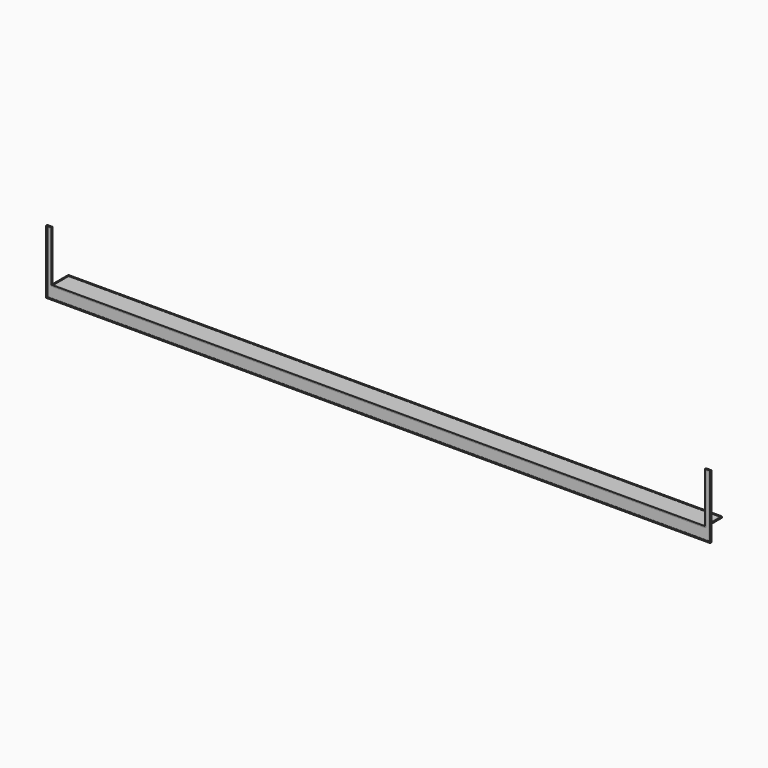
from build123d import *

# Parameters (mm, degrees)
F1_DEPTH     = 3.175
F3_W         = 1562.1
F3_H         = 50.8
F4_DEPTH     = 3.175
F5_T         = 2.54
F5_T3_DEPTH  = 8.255
F5_T5_DEPTH  = 1567.18
F6_T         = 2.54
F6_T3_DEPTH  = 8.255
F6_T5_DEPTH  = 8.255
F6_T7_DEPTH  = 1567.18
F6_T9_DEPTH  = 5.715
F6_T11_DEPTH = 50.165
F6_T13_DEPTH = 5.715
F6_T15_DEPTH = 1562.1


# Not quite as in the source:
# - a shell that OpenCascade refuses in one call is made with other operations: the cavity is built on its own and cut out


with BuildPart() as f1:
    # F0 (on Front) → F1 (new body)
    with BuildSketch(Plane.XZ):
        Polygon((-781.05, 156.1854919385), (-793.75, 156.1854919385), (-793.75, 3.7854919385), (793.75, 3.7854919385), (793.75, 156.1854919385), (781.05, 156.1854919385), (781.05, 35.5354919385), (-781.05, 35.5354919385), align=None)
    extrude(amount=F1_DEPTH)

    # F3 (on face) → F4 (join)
    with BuildSketch(Plane.XY.offset(35.5354919385)):
        with Locations((0, 22.225)):
            Rectangle(F3_W, F3_H)
    extrude(amount=-F4_DEPTH)

    # F5: shell of thickness 2.54, made by hand


with BuildPart() as f5_core1:
    # F5_t2: copy of F1
    add(f1.part)

    # the walls: a layer under each face that stays
    f5_faces = [f5_core1.faces().sort_by_distance(p)[0] for p in [
        (-781.05, -1.5875, 95.8604919385),
        (-787.4, -1.5875, 156.1854919385),
        (-529.1666666667, 0, 29.1854919385),
        (-529.1666666667, -3.175, 29.1854919385),
        (781.05, -1.5875, 95.8604919385),
        (-793.75, -1.5875, 79.9854919385),
        (-781.05, 23.8125, 33.9479919385),
        (0, 23.8125, 32.3604919385),
        (781.05, 23.8125, 33.9479919385),
        (787.4, -1.5875, 156.1854919385),
        (793.75, -1.5875, 79.9854919385),
        (0, -1.5875, 3.7854919385),
        (0, 47.625, 33.9479919385),
    ]]
    thicken(f5_faces, amount=-F5_T, mode=Mode.SUBTRACT)

    # F5_s4 → F5_t3 (cut)
    with BuildSketch(Plane.XY.offset(29.8204919385)):
        Polygon((-781.0754, 0.0254), (-781.05, -2.54), (-778.51, -2.54), (-778.51, 0), align=None)
        Polygon((781.0754, 0.0254), (781.05, -2.54), (778.51, -2.54), (778.51, 0), align=None)
    extrude(amount=F5_T3_DEPTH, mode=Mode.SUBTRACT)

    # F5_s6 → F5_t5 (cut)
    with BuildSketch(Plane.YZ.offset(-783.59)):
        Polygon((0.0254, 32.3350919385), (-2.54, 32.3604919385), (-2.54, 34.9004919385), (0, 34.9004919385), align=None)
    extrude(amount=F5_T5_DEPTH, mode=Mode.SUBTRACT)


with BuildPart() as f1_1:
    add(f1.part)

    # what is left inside the walls is the cavity
    f5_cavity = [f5_core1.part.solids().sort_by_distance(p)[0] for p in [
        (0, 14.605, 34.925892),
    ]]
    add(f5_cavity, mode=Mode.SUBTRACT)

    # F6: shell of thickness 2.54, made by hand


with BuildPart() as f6_core1:
    # F6_t2: copy of F1
    add(f1_1.part)

    # the walls: a layer under each face that stays
    f6_faces = [f6_core1.faces().sort_by_distance(p)[0] for p in [
        (-781.05, -1.5875, 95.8604919385),
        (728.98, -1.4816666667, 35.5354919385),
        (-787.4, -1.5875, 156.1854919385),
        (-529.1666666667, 0, 29.1854919385),
        (781.05, -1.5875, 95.8604919385),
        (781.05, 23.8125, 33.9479919385),
        (0, 47.625, 33.9479919385),
        (-781.05, 23.8125, 33.9479919385),
        (778.51, 22.225, 35.2179919385),
        (0, -0.635, 35.2179919385),
        (-778.51, 22.225, 35.2179919385),
        (0, 45.085, 35.2179919385),
        (-793.75, -1.5875, 79.9854919385),
        (0, 23.8125, 32.3604919385),
        (787.4, -1.5875, 156.1854919385),
        (793.75, -1.5875, 79.9854919385),
        (0, -1.5875, 3.7854919385),
        (0, 22.225, 34.9004919385),
    ]]
    thicken(f6_faces, amount=-F6_T, mode=Mode.SUBTRACT)

    # F6_s4 → F6_t3 (cut)
    with BuildSketch(Plane.XZ.offset(-2.54)):
        Polygon((-781.0246, 35.5608919385), (-783.59, 35.5354919385), (-783.59, 32.9954919385), (-781.05, 32.9954919385), align=None)
        Polygon((781.0246, 35.5608919385), (781.05, 32.9954919385), (783.59, 32.9954919385), (783.59, 35.5354919385), align=None)
    extrude(amount=F6_T3_DEPTH, mode=Mode.SUBTRACT)

    # F6_s6 → F6_t5 (cut)
    with BuildSketch(Plane.XY.offset(29.8204919385)):
        Polygon((-781.0754, 0.0254), (-781.05, -2.54), (-778.51, -2.54), (-778.51, 0), align=None)
        Polygon((781.0754, 0.0254), (781.05, -2.54), (778.51, -2.54), (778.51, 0), align=None)
    extrude(amount=F6_T5_DEPTH, mode=Mode.SUBTRACT)

    # F6_s8 → F6_t7 (cut)
    with BuildSketch(Plane.YZ.offset(-783.59)):
        Polygon((0.0254, 32.3350919385), (-2.54, 32.3604919385), (-2.54, 34.9004919385), (0, 34.9004919385), align=None)
    extrude(amount=F6_T7_DEPTH, mode=Mode.SUBTRACT)

    # F6_s10 → F6_t9 (cut)
    with BuildSketch(Plane.XY.offset(32.3604919385)):
        Polygon((778.4846, 45.0596), (781.05, 45.085), (781.05, 47.625), (778.51, 47.625), align=None)
        Polygon((778.4846, -0.6096), (781.05, -0.635), (781.05, -3.175), (778.51, -3.175), align=None)
        Polygon((-778.4846, -0.6096), (-778.51, -3.175), (-781.05, -3.175), (-781.05, -0.635), align=None)
        Polygon((-778.4846, 45.0596), (-781.05, 45.085), (-781.05, 47.625), (-778.51, 47.625), align=None)
    extrude(amount=F6_T9_DEPTH, mode=Mode.SUBTRACT)

    # F6_s12 → F6_t11 (cut)
    with BuildSketch(Plane.XZ.offset(-47.625)):
        Polygon((778.4846, 34.9258919385), (781.05, 34.9004919385), (781.05, 32.3604919385), (778.51, 32.3604919385), align=None)
        Polygon((-778.4846, 34.9258919385), (-781.05, 34.9004919385), (-781.05, 32.3604919385), (-778.51, 32.3604919385), align=None)
    extrude(amount=F6_T11_DEPTH, mode=Mode.SUBTRACT)

    # F6_s14 → F6_t13 (cut)
    with BuildSketch(Plane.XZ.offset(-2.54)):
        Polygon((778.4846, 34.9258919385), (781.05, 34.9004919385), (781.05, 32.3604919385), (778.51, 32.3604919385), align=None)
        Polygon((-778.4846, 34.9258919385), (-781.05, 34.9004919385), (-781.05, 32.3604919385), (-778.51, 32.3604919385), align=None)
    extrude(amount=F6_T13_DEPTH, mode=Mode.SUBTRACT)

    # F6_s16 → F6_t15 (cut)
    with BuildSketch(Plane.YZ.offset(-781.05)):
        Polygon((-0.6096, 34.9258919385), (-3.175, 34.9004919385), (-3.175, 32.3604919385), (-0.635, 32.3604919385), align=None)
        Polygon((45.0596, 34.9258919385), (47.625, 34.9004919385), (47.625, 32.3604919385), (45.085, 32.3604919385), align=None)
    extrude(amount=F6_T15_DEPTH, mode=Mode.SUBTRACT)


with BuildPart() as f1_2:
    add(f1_1.part)

    # what is left inside the walls is the cavity
    f6_cavity = [f6_core1.part.solids().sort_by_distance(p)[0] for p in [
        (395.605, -2.5654, 22.694381),
    ]]
    add(f6_cavity, mode=Mode.SUBTRACT)


solid = f1_2.part
